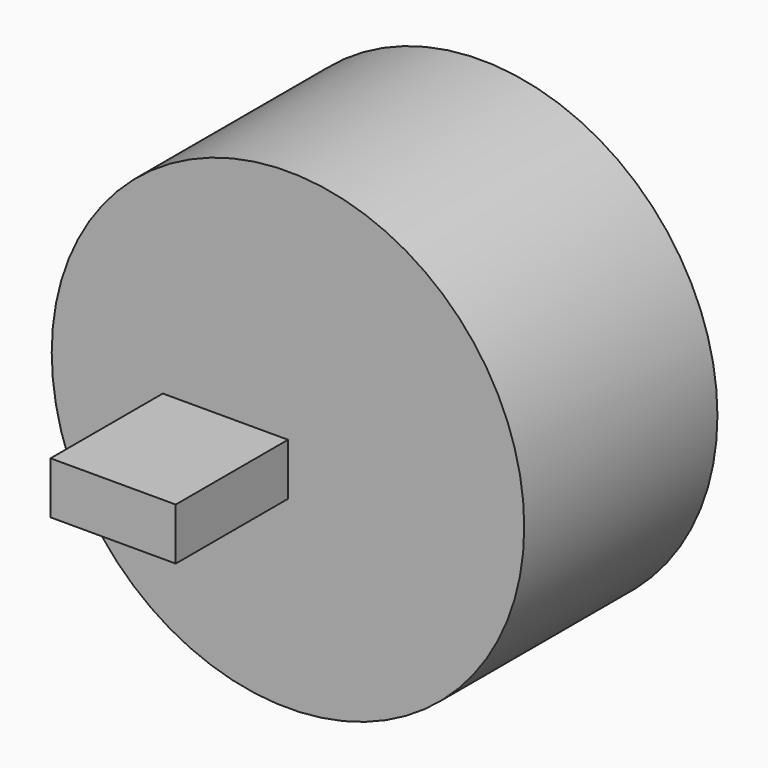
from build123d import *

# Parameters (mm, degrees)
F0_W     = 61.1385069788
F0_H     = 68.5273110867
F1_DEPTH = 25.4
F2_W     = 115.3954155743
F2_H     = 117.9477572441


# Not quite as in the source:
# - the program builds the solid bodies; features that only make, move or delete a surface that nothing else refers to are left out


with BuildPart() as f1:
    # F0 (on Top) → F1 (new body)
    with BuildSketch(Plane.XY):
        with Locations((30.5692534894, 34.2636555433)):
            Rectangle(F0_W, F0_H)
    extrude(amount=F1_DEPTH)

    # F2 (on face) → F4 (revolve)
    with BuildSketch(Plane.XY.offset(25.4)):
        with Locations((118.8362147659, 127.5011897087)):
            Rectangle(F2_W, F2_H)
    revolve(axis=Axis((61.1385069788, 34.2636555433, 25.4), (0, -1, 0)))


solid = f1.part
